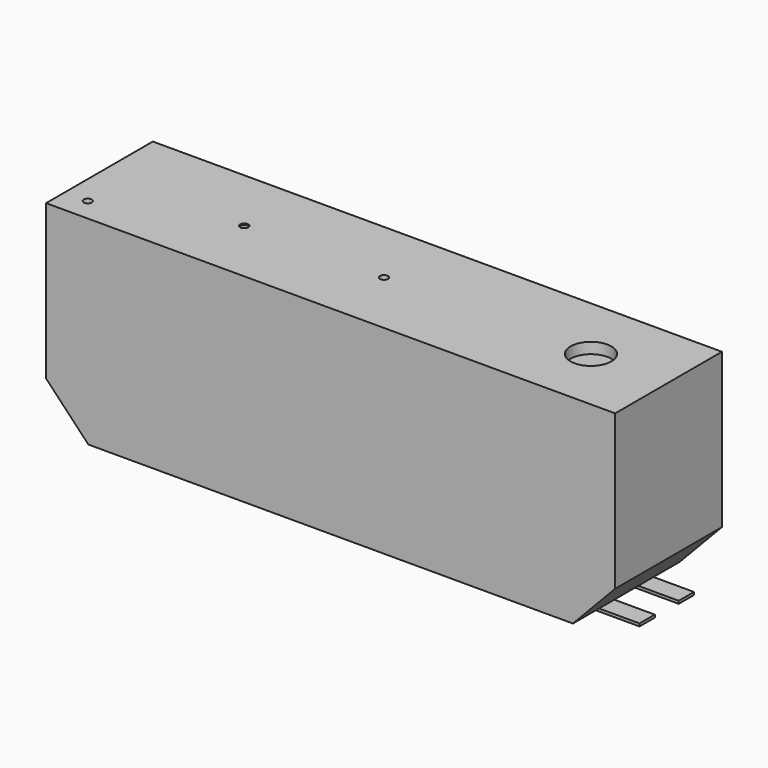
from build123d import *

# Parameters (mm, degrees)
F0_W      = 1320.8
F0_H      = 457.2
F1_DEPTH  = 152.4
F2_R      = 50.8
F2_R_2    = 12.7
F3_DEPTH  = 25.4
F6_DEPTH  = 304.8
F7_T      = 3.175
F8_W      = 152.4
F8_H      = 44.45
F9_DEPTH  = 6.35
F11_R     = 9.525
F12_DEPTH = 12.7
F10_R     = 12.7
F13_DEPTH = 12.7


with BuildPart() as f1:
    # F0 (on Front) → F1 (new body, symmetric)
    with BuildSketch(Plane.XZ):
        Rectangle(F0_W, F0_H)
    extrude(amount=F1_DEPTH, both=True)

    # F2 (on face) → F3 (cut, symmetric)
    with BuildSketch(Plane.XY.offset(228.6)):
        with Locations((482.6, 0)):
            Circle(F2_R)
        Circle(F2_R_2)
        with Locations((-609.6, -101.6)):
            Circle(F2_R_2)
    extrude(amount=F3_DEPTH, both=True, mode=Mode.SUBTRACT)

    # F5 (on face) → F6 (cut, through all)
    with BuildSketch(Plane.XZ.offset(152.4)):
        Polygon((-559.0197953224, -233.4262882042), (-660.6197953224, -126.7462882042), (-660.6197953224, -233.4262882042), align=None)
        Polygon((660.6197953224, -126.7462882042), (559.0197953224, -233.4262882042), (660.6197953224, -233.4262882042), align=None)
    extrude(amount=-F6_DEPTH, mode=Mode.SUBTRACT)

    # F7 (hollow, outwards: the wall grows on the outside; the body as it was is the cavity)
    f7_inside = f1.part
    offset(amount=F7_T, kind=Kind.INTERSECTION)
    add(f7_inside, mode=Mode.SUBTRACT)

    # F8 (on face) → F9 (join)
    with BuildSketch(Plane(origin=(0, 0, -231.775), x_dir=(1, 0, 0), z_dir=(0, 0, -1))):
        with Locations((583.1482922554, -57.15)):
            Rectangle(F8_W, F8_H)
        with Locations((583.1482922554, 57.15)):
            Rectangle(F8_W, F8_H)
    extrude(amount=F9_DEPTH)

    # F11 (on face) → F12 (cut, symmetric)
    with BuildSketch(Plane.XY.offset(231.775)):
        with Locations((-325.7964868545, 0)):
            Circle(F11_R)
    extrude(amount=F12_DEPTH, both=True, mode=Mode.SUBTRACT)

    # F10 (on face) → F13 (cut, symmetric)
    with BuildSketch(Plane(origin=(0, 0, -231.775), x_dir=(1, 0, 0), z_dir=(0, 0, -1))):
        Circle(F10_R)
    extrude(amount=F13_DEPTH, both=True, mode=Mode.SUBTRACT)


solid = f1.part
